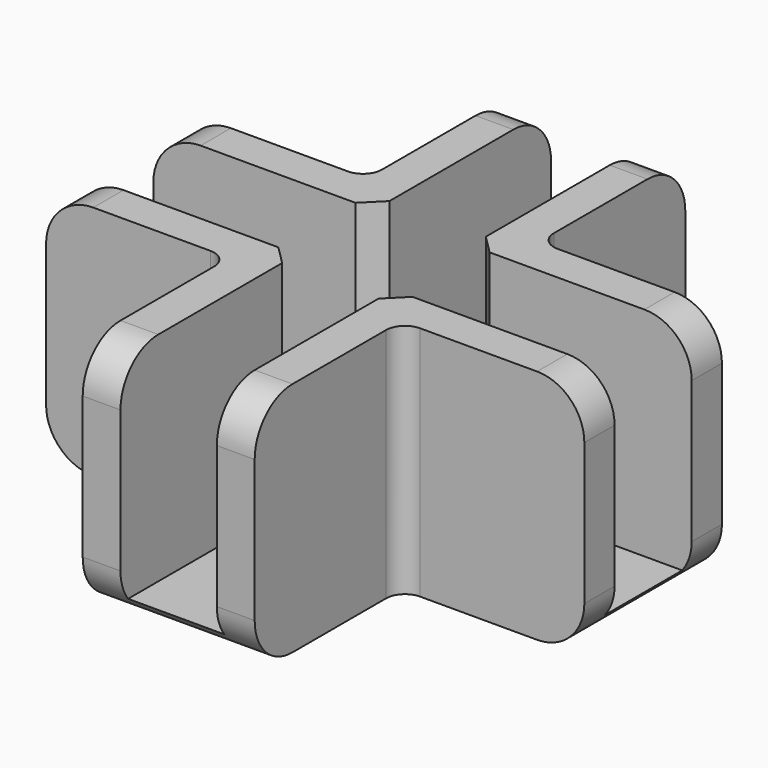
from build123d import *

# Parameters (mm, degrees)
F1_DEPTH       = 2
F2_DEPTH       = 25
F3_R           = 2
F4_T1_DEPTH    = 4
F4_T3_DEPTH    = 4
F4_T5_DEPTH    = 4
F4_T7_DEPTH    = 18.2
F4_T9_DEPTH    = 18.2
F4_T11_DEPTH   = 4
F5_R           = 2
F6_SIZE        = 2
F8_D           = 3.3
F8_CSINK_D     = 6
F8_CSINK_ANGLE = 90


# Not quite as in the source:
# - a fillet or chamfer that OpenCascade refuses, or shapes differently, is made with other operations: its cross-section is extruded or revolved along the edge and cut away or added
# - a feature names something its author has since deleted; it is built from what else it names


with BuildPart() as f1:
    # F0 (on Top) → F1 (new body)
    with BuildSketch(Plane.XY):
        Polygon((28.4836267311, 0), (28.4836267311, 10.2), (5.1, 10.2), (5.1, 33.5836267311), (-5.1, 33.5836267311), (-5.1, 10.2), (-28.4836267311, 10.2), (-28.4836267311, 0), (-5.1, 0), (-5.1, -23.3836267311), (5.1, -23.3836267311), (5.1, 0), align=None)
        Polygon((5.1, 10.2), (28.4836267311, 10.2), (28.4836267311, 14.2), (9.1, 14.2), (9.1, 33.5836267311), (5.1, 33.5836267311), align=None)
        Polygon((28.4836267311, -4), (28.4836267311, 0), (5.1, 0), (5.1, -23.3836267311), (9.1, -23.3836267311), (9.1, -4), align=None)
        Polygon((-5.1, 10.2), (-5.1, 33.5836267311), (-9.1, 33.5836267311), (-9.1, 14.2), (-28.4836267311, 14.2), (-28.4836267311, 10.2), align=None)
        Polygon((-9.1, -23.3836267311), (-5.1, -23.3836267311), (-5.1, 0), (-28.4836267311, 0), (-28.4836267311, -4), (-9.1, -4), align=None)
    extrude(amount=F1_DEPTH)

    # F0 (on Top) → F2 (join)
    with BuildSketch(Plane.XY):
        Polygon((-5.1, 10.2), (-5.1, 33.5836267311), (-9.1, 33.5836267311), (-9.1, 14.2), (-28.4836267311, 14.2), (-28.4836267311, 10.2), align=None)
        Polygon((5.1, 10.2), (28.4836267311, 10.2), (28.4836267311, 14.2), (9.1, 14.2), (9.1, 33.5836267311), (5.1, 33.5836267311), align=None)
        Polygon((-9.1, -23.3836267311), (-5.1, -23.3836267311), (-5.1, 0), (-28.4836267311, 0), (-28.4836267311, -4), (-9.1, -4), align=None)
        Polygon((28.4836267311, -4), (28.4836267311, 0), (5.1, 0), (5.1, -23.3836267311), (9.1, -23.3836267311), (9.1, -4), align=None)
    extrude(amount=F2_DEPTH)

    # F3
    f3_edges = [f1.edges().sort_by_distance(p)[0] for p in [
        (9.1, 14.2, 12.5),
        (9.1, -4, 12.5),
    ]]
    fillet(f3_edges, radius=F3_R)

    # F4: fillet of radius 5 on 12 edges, made by hand

    # F4_s2 → F4_t1 (cut)
    with BuildSketch(Plane.XZ.offset(-14.2)):
        with BuildLine():
            ThreePointArc((23.4836267311, 25), (27.0191606371, 23.5355339059), (28.4836267311, 20))
            Line((28.4836267311, 20), (28.5836267311, 20))
            Line((28.5836267311, 20), (28.5836267311, 25.1))
            Line((28.5836267311, 25.1), (23.4836267311, 25.1))
            Line((23.4836267311, 25.1), (23.4836267311, 25))
        make_face()
        with BuildLine():
            ThreePointArc((-28.4836267311, 20), (-27.0191606371, 23.5355339059), (-23.4836267311, 25))
            Line((-23.4836267311, 25), (-23.4836267311, 25.1))
            Line((-23.4836267311, 25.1), (-28.5836267311, 25.1))
            Line((-28.5836267311, 25.1), (-28.5836267311, 20))
            Line((-28.5836267311, 20), (-28.4836267311, 20))
        make_face()
    extrude(amount=F4_T1_DEPTH, mode=Mode.SUBTRACT)

    # F4_s4 → F4_t3 (cut)
    with BuildSketch(Plane.YZ.offset(-9.1)):
        with BuildLine():
            ThreePointArc((33.5836267311, 20), (32.1191606371, 23.5355339059), (28.5836267311, 25))
            Line((28.5836267311, 25), (28.5836267311, 25.1))
            Line((28.5836267311, 25.1), (33.6836267311, 25.1))
            Line((33.6836267311, 25.1), (33.6836267311, 20))
            Line((33.6836267311, 20), (33.5836267311, 20))
        make_face()
        with BuildLine():
            ThreePointArc((-23.3836267311, 20), (-21.9191606371, 23.5355339059), (-18.3836267311, 25))
            Line((-18.3836267311, 25), (-18.3836267311, 25.1))
            Line((-18.3836267311, 25.1), (-23.4836267311, 25.1))
            Line((-23.4836267311, 25.1), (-23.4836267311, 20))
            Line((-23.4836267311, 20), (-23.3836267311, 20))
        make_face()
    extrude(amount=F4_T3_DEPTH, mode=Mode.SUBTRACT)

    # F4_s6 → F4_t5 (cut)
    with BuildSketch(Plane.YZ.offset(5.1)):
        with BuildLine():
            ThreePointArc((28.5836267311, 25), (32.1191606371, 23.5355339059), (33.5836267311, 20))
            Line((33.5836267311, 20), (33.6836267311, 20))
            Line((33.6836267311, 20), (33.6836267311, 25.1))
            Line((33.6836267311, 25.1), (28.5836267311, 25.1))
            Line((28.5836267311, 25.1), (28.5836267311, 25))
        make_face()
        with BuildLine():
            ThreePointArc((-18.3836267311, 25), (-21.9191606371, 23.5355339059), (-23.3836267311, 20))
            Line((-23.3836267311, 20), (-23.4836267311, 20))
            Line((-23.4836267311, 20), (-23.4836267311, 25.1))
            Line((-23.4836267311, 25.1), (-18.3836267311, 25.1))
            Line((-18.3836267311, 25.1), (-18.3836267311, 25))
        make_face()
    extrude(amount=F4_T5_DEPTH, mode=Mode.SUBTRACT)

    # F4_s8 → F4_t7 (cut)
    with BuildSketch(Plane.XZ.offset(-14.2)):
        with BuildLine():
            ThreePointArc((-23.4836267311, 0), (-27.0191606371, 1.4644660941), (-28.4836267311, 5))
            Line((-28.4836267311, 5), (-28.5836267311, 5))
            Line((-28.5836267311, 5), (-28.5836267311, -0.1))
            Line((-28.5836267311, -0.1), (-23.4836267311, -0.1))
            Line((-23.4836267311, -0.1), (-23.4836267311, 0))
        make_face()
        with BuildLine():
            ThreePointArc((28.4836267311, 5), (27.0191606371, 1.4644660941), (23.4836267311, 0))
            Line((23.4836267311, 0), (23.4836267311, -0.1))
            Line((23.4836267311, -0.1), (28.5836267311, -0.1))
            Line((28.5836267311, -0.1), (28.5836267311, 5))
            Line((28.5836267311, 5), (28.4836267311, 5))
        make_face()
    extrude(amount=F4_T7_DEPTH, mode=Mode.SUBTRACT)

    # F4_s10 → F4_t9 (cut)
    with BuildSketch(Plane.YZ.offset(-9.1)):
        with BuildLine():
            ThreePointArc((28.5836267311, 0), (32.1191606371, 1.4644660941), (33.5836267311, 5))
            Line((33.5836267311, 5), (33.6836267311, 5))
            Line((33.6836267311, 5), (33.6836267311, -0.1))
            Line((33.6836267311, -0.1), (28.5836267311, -0.1))
            Line((28.5836267311, -0.1), (28.5836267311, 0))
        make_face()
        with BuildLine():
            ThreePointArc((-18.3836267311, 0), (-21.9191606371, 1.4644660941), (-23.3836267311, 5))
            Line((-23.3836267311, 5), (-23.4836267311, 5))
            Line((-23.4836267311, 5), (-23.4836267311, -0.1))
            Line((-23.4836267311, -0.1), (-18.3836267311, -0.1))
            Line((-18.3836267311, -0.1), (-18.3836267311, 0))
        make_face()
    extrude(amount=F4_T9_DEPTH, mode=Mode.SUBTRACT)

    # F4_s12 → F4_t11 (cut)
    with BuildSketch(Plane.XZ):
        with BuildLine():
            ThreePointArc((28.4836267311, 20), (27.0191606371, 23.5355339059), (23.4836267311, 25))
            Line((23.4836267311, 25), (23.4836267311, 25.1))
            Line((23.4836267311, 25.1), (28.5836267311, 25.1))
            Line((28.5836267311, 25.1), (28.5836267311, 20))
            Line((28.5836267311, 20), (28.4836267311, 20))
        make_face()
        with BuildLine():
            ThreePointArc((-28.4836267311, 20), (-27.0191606371, 23.5355339059), (-23.4836267311, 25))
            Line((-23.4836267311, 25), (-23.4836267311, 25.1))
            Line((-23.4836267311, 25.1), (-28.5836267311, 25.1))
            Line((-28.5836267311, 25.1), (-28.5836267311, 20))
            Line((-28.5836267311, 20), (-28.4836267311, 20))
        make_face()
    extrude(amount=F4_T11_DEPTH, mode=Mode.SUBTRACT)

    # F5
    f5_edges = [f1.edges().sort_by_distance(p)[0] for p in [
        (-9.1, 14.2, 12.5),
        (-9.1, -4, 12.5),
    ]]
    fillet(f5_edges, radius=F5_R)

    # F6
    f6_edges = [f1.edges().sort_by_distance(p)[0] for p in [
        (5.1, 10.2, 13.5),
        (-5.1, 10.2, 13.5),
        (5.1, 0, 13.5),
        (-5.1, 0, 13.5),
    ]]
    chamfer(f6_edges, length=F6_SIZE)

    # F8 (through all)
    with Locations(Plane(origin=(0, 0, 0), x_dir=(1, 0, 0), z_dir=(0, 0, -1))):
        with Locations((0, 9.587961331), (-15, -5.1), (15, -5.1), (0, -20.1)):
            CounterSinkHole(F8_D / 2, F8_CSINK_D / 2, counter_sink_angle=F8_CSINK_ANGLE)


solid = f1.part
